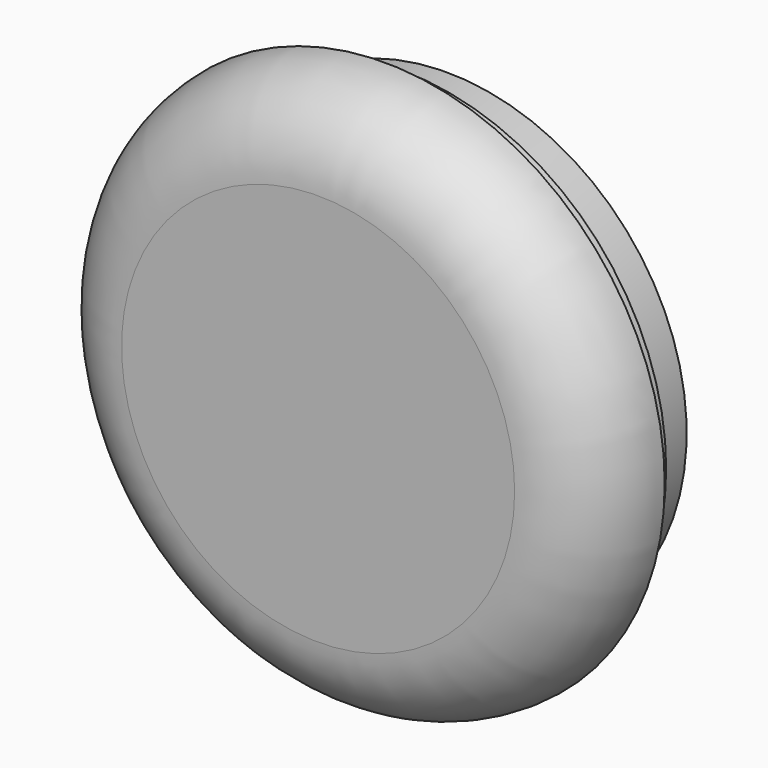
from build123d import *

# Parameters (mm, degrees)
F0_R     = 17.0561
F1_DEPTH = 5.08
F2_R     = 16.129
F3_DEPTH = 1.27
F4_R     = 5.07999
F5_R     = 14.605
F6_DEPTH = 3.4642005339


# Not quite as in the source:
# - a fillet or chamfer is up to 0.001 mm smaller than in the source, because OpenCascade refuses the exact size


with BuildPart() as f1:
    # F0 (on Front) → F1 (new body)
    with BuildSketch(Plane.XZ):
        Circle(F0_R)
    extrude(amount=-F1_DEPTH)

    # F2 (on face) → F3 (join)
    with BuildSketch(Plane(origin=(0, 5.08, 0), x_dir=(-1, 0, 0), z_dir=(0, 1, 0))):
        Circle(F2_R)
    extrude(amount=F3_DEPTH)

    # F4 (radius 5.08 in the source; OpenCascade refuses exactly that, so slightly less here)
    f4_edges = [f1.edges().sort_by_distance(p)[0] for p in [
        (-17.0561, 0, 0),
    ]]
    fillet(f4_edges, radius=F4_R)

    # F5 (on face) → F6 (join)
    with BuildSketch(Plane(origin=(0, 6.35, 0), x_dir=(-1, 0, 0), z_dir=(0, 1, 0))):
        Circle(F5_R)
    extrude(amount=F6_DEPTH)


solid = f1.part
